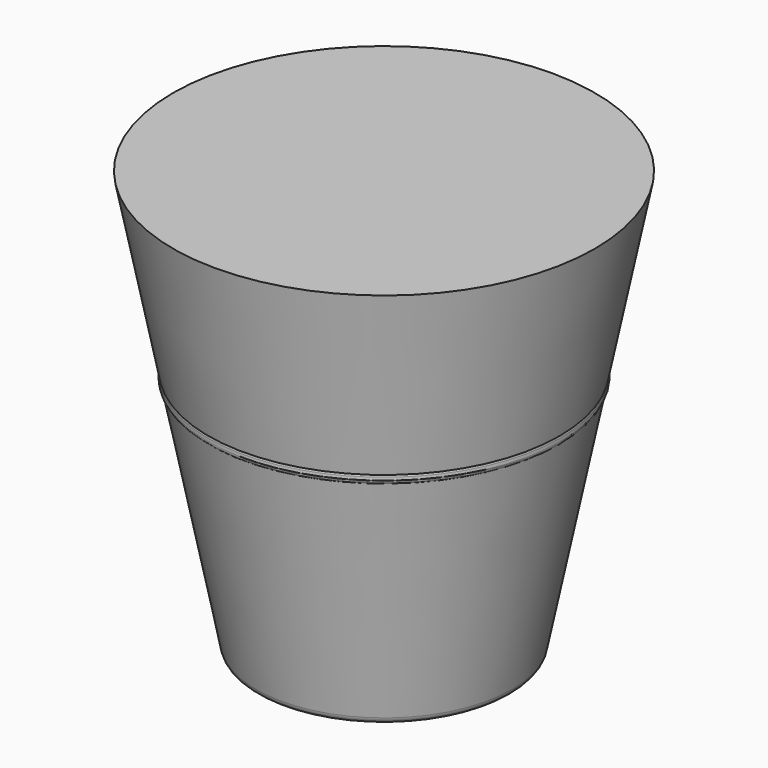
from build123d import *

# Parameters (mm, degrees)
F2_R = 1


# Not quite as in the source:
# - a fillet or chamfer that OpenCascade refuses, or shapes differently, is made with other operations: its cross-section is extruded or revolved along the edge and cut away or added


with BuildPart() as f1:
    # F0 (on Front) → F1 (revolve)
    with BuildSketch(Plane.XZ):
        Polygon((0, 50), (0, 0), (15, 0), (20.62, 28.1), (20.82, 29.1), (25, 50), align=None)
        Polygon((20.82, 29.1), (20.62, 28.1), (20.87, 28.1), (20.87, 29.1), align=None)
    revolve(axis=Axis((0, 0, 25), (0, 0, -1)))

    # F2
    f2_edges = [f1.edges().sort_by_distance(p)[0] for p in [
        (-15, 0, 0),
    ]]
    fillet(f2_edges, radius=F2_R)

    # F3: fillet of radius 0.5 on 2 edges, made by hand

    # F3_s1 → F3_t2 (revolve, cut)
    with BuildSketch(Plane.XZ):
        with BuildLine():
            ThreePointArc((20.62, 28.1), (20.8030127019, 28.2830127019), (20.87, 28.5330127019))
            Line((20.87, 28.5330127019), (20.88, 28.5330127019))
            Line((20.88, 28.5330127019), (20.88, 28.1))
            Line((20.88, 28.1), (20.87, 28.09))
            ThreePointArc((20.87, 28.09), (20.745, 28.09), (20.625, 28.091339746))
            Line((20.625, 28.091339746), (20.62, 28.1))
        make_face()
    revolve(axis=Axis((0, 0, 28.1), (0, 0, -1)), mode=Mode.SUBTRACT)

    # F3_s3 → F3_t4 (revolve, cut)
    with BuildSketch(Plane.XZ):
        with BuildLine():
            ThreePointArc((20.87, 28.8820550528), (20.8573397172, 28.9938584517), (20.82, 29.1))
            Line((20.82, 29.1), (20.829, 29.1043588989))
            ThreePointArc((20.829, 29.1043588989), (20.845, 29.11), (20.87, 29.11))
            Line((20.87, 29.11), (20.88, 29.1))
            Line((20.88, 29.1), (20.88, 28.8820550528))
            Line((20.88, 28.8820550528), (20.87, 28.8820550528))
        make_face()
    revolve(axis=Axis((0, 0, 29.1), (0, 0, -1)), mode=Mode.SUBTRACT)


solid = f1.part
